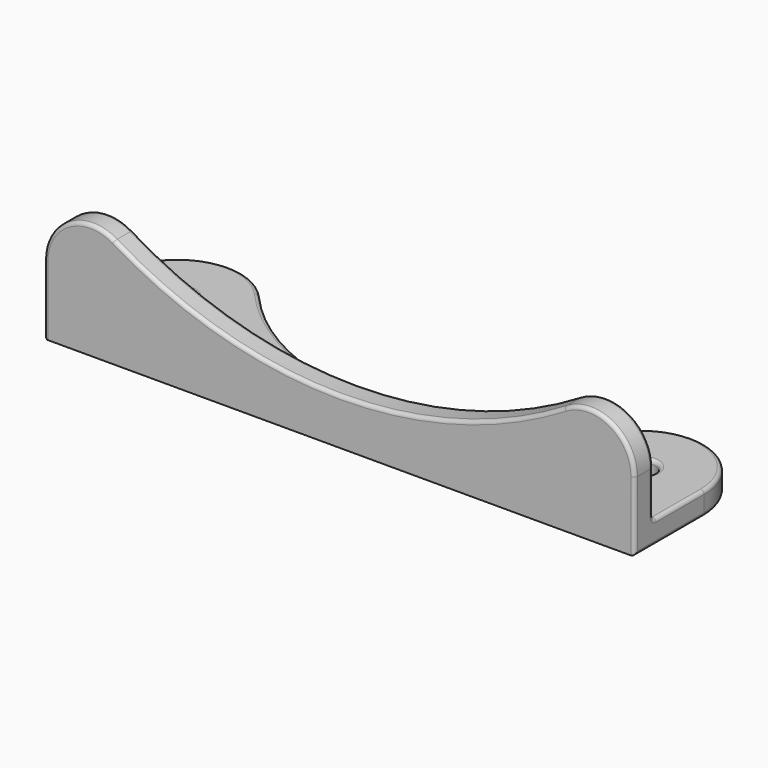
from build123d import *

# Parameters (mm, degrees)
F1_DEPTH = 6.35
F2_W     = 162
F2_H     = 6.35
F3_DEPTH = 41.35
F5_D     = 8
F7_DEPTH = 6.35
F8_R     = 1


with BuildPart() as f1:
    # F0 (on Top) → F1 (new body)
    with BuildSketch(Plane.XY):
        with BuildLine():
            ThreePointArc((17.5, 0), (29.8743686708, 5.1256313292), (35, 17.5))
            ThreePointArc((35, 17.5), (33.8685421385, 23.6903819156), (30.6204767701, 29.0802888273))
            ThreePointArc((30.6204767701, 29.0802888273), (11.3096180844, 33.8685421385), (0, 17.5))
            ThreePointArc((0, 17.5), (5.1256313292, 5.1256313292), (17.5, 0))
        make_face()
        with BuildLine():
            Line((0, 0), (17.5, 0))
            ThreePointArc((17.5, 0), (5.1256313292, 5.1256313292), (0, 17.5))
            Line((0, 17.5), (0, 0))
        make_face()
        with BuildLine():
            ThreePointArc((30.6204767701, 29.0802888273), (33.8685421385, 23.6903819156), (35, 17.5))
            ThreePointArc((35, 17.5), (29.8743686708, 5.1256313292), (17.5, 0))
            Line((17.5, 0), (144.5, 0))
            ThreePointArc((144.5, 0), (128.5484318251, 10.3029538864), (131.3795232299, 29.0802888273))
            ThreePointArc((131.3795232299, 29.0802888273), (81, 6.35), (30.6204767701, 29.0802888273))
        make_face()
        with BuildLine():
            ThreePointArc((162, 17.5), (150.6903819156, 33.8685421385), (131.3795232299, 29.0802888273))
            ThreePointArc((131.3795232299, 29.0802888273), (128.5484318251, 10.3029538864), (144.5, 0))
            ThreePointArc((144.5, 0), (156.8743686708, 5.1256313292), (162, 17.5))
        make_face()
        with BuildLine():
            ThreePointArc((162, 17.5), (156.8743686708, 5.1256313292), (144.5, 0))
            Line((144.5, 0), (162, 0))
            Line((162, 0), (162, 17.5))
        make_face()
    extrude(amount=-F1_DEPTH)

    # F2 (on face) → F3 (join)
    with BuildSketch(Plane(origin=(0, 0, -6.35), x_dir=(1, 0, 0), z_dir=(0, 0, -1))):
        with Locations((81, 3.175)):
            Rectangle(F2_W, F2_H)
    extrude(amount=-F3_DEPTH)

    # F5 (through all)
    with Locations(Plane.XY):
        with Locations((17.5, 17.5), (144.5, 17.5)):
            Hole(F5_D / 2)

    # F6 (on face) → F7 (cut, through all)
    with BuildSketch(Plane(origin=(0, 0, 0), x_dir=(-1, 0, 0), z_dir=(0, 1, 0))):
        with BuildLine():
            ThreePointArc((-19.273127471, 23.5666459982), (-6.4625613783, 23.7627464691), (0, 12.7))
            Line((0, 12.7), (0, 35))
            Line((0, 35), (-162, 35))
            Line((-162, 35), (-162, 12.7))
            ThreePointArc((-162, 12.7), (-155.5374386217, 23.7627464691), (-142.726872529, 23.5666459982))
            ThreePointArc((-142.726872529, 23.5666459982), (-81, 6.35), (-19.273127471, 23.5666459982))
        make_face()
    extrude(amount=-F7_DEPTH, mode=Mode.SUBTRACT)

    # F8
    f8_edges = [f1.edges().sort_by_distance(p)[0] for p in [
        (150.690382, 33.868542, 0),
        (81, 0, 0),
        (11.309618, 33.868542, -6.35),
        (6.462561, -6.35, 23.762746),
        (11.309618, 33.868542, 0),
        (81, 6.35, 0),
        (81, 6.35, -6.35),
        (0, 8.75, 0),
        (0, 0, 6.35),
        (0, -6.35, 3.175),
        (0, 5.575, -6.35),
        (162, 8.75, 0),
        (13.5, 17.5, 0),
        (140.5, 17.5, 0),
        (150.690382, 33.868542, -6.35),
        (162, 5.575, -6.35),
        (13.5, 17.5, -6.35),
        (140.5, 17.5, -6.35),
        (162, 0, 6.35),
        (155.537439, 0, 23.762746),
        (81, 0, 6.35),
        (6.462561, 0, 23.762746),
        (81, -6.35, 6.35),
        (155.537439, -6.35, 23.762746),
        (162, -6.35, 3.175),
    ]]
    fillet(f8_edges, radius=F8_R)


solid = f1.part
